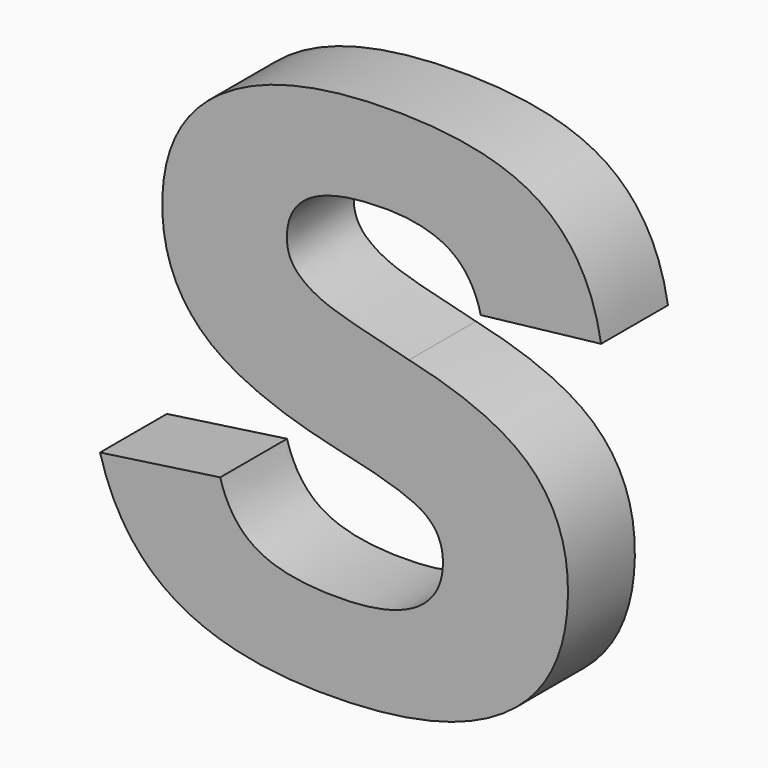
from build123d import *

# Parameters (mm, degrees)
F0_TEXT_SIZE = 58.6762183553
F1_DEPTH     = 5


# Not quite as in the source:
# - Text() gives the source's letters only with a copy of the font that has no kerning and outlines rounded to 1/6400 em; it was checked with that copy


with BuildPart() as f1:
    # F0 (on Front) → F1 (new body)
    with BuildSketch(Plane.XZ):
        with Locations((-63.5858550668, -7.9751750454)):
            Text('s', F0_TEXT_SIZE, font='Arimo', font_style=FontStyle.BOLDITALIC, text_align=(TextAlign.LEFT, TextAlign.BOTTOM))
    extrude(amount=F1_DEPTH)


solid = f1.part
